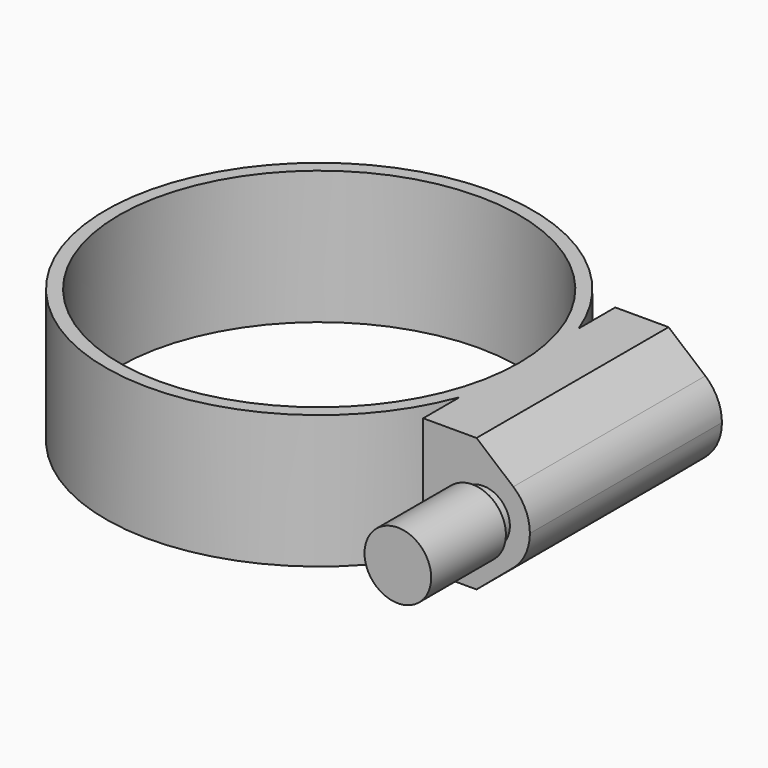
from build123d import *

# Parameters (mm, degrees)
F4_DEPTH      = 9
F4_DEPTH_BACK = 9


with BuildPart() as f3:
    # F2 (on plane+point) → F3 (revolve)
    with BuildSketch(Plane.XY.offset(5)):
        Polygon((19.5, -17), (19.5, 11), (18.5, 11), (17.5, 10), (17.5, -10), (17, -10), (17, -17), align=None)
    revolve(axis=Axis((19.5, -3, 5), (0, -1, 0)))

    # F0 (on Front) → F4 (join, two sides)
    with BuildSketch(Plane.XZ) as f4_sk:
        Polygon((15, 10), (15, 0), (16, 0), (16, 5), (16, 10), align=None)
        with BuildLine():
            Line((16, 10), (16, 5))
            ThreePointArc((16, 5), (18.024725, 8.173888), (21.756323, 7.675632))
            Line((21.756323, 7.675632), (19, 10))
            Line((19, 10), (16, 10))
        make_face()
        with BuildLine():
            Line((16, 5), (16, 0))
            Line((16, 0), (19, 0))
            Line((19, 0), (21.756323, 2.324368))
            ThreePointArc((21.756323, 2.324368), (18.024725, 1.826112), (16, 5))
        make_face()
        with BuildLine():
            ThreePointArc((21.756323, 7.675632), (18.024725, 8.173888), (16, 5))
            ThreePointArc((16, 5), (18.024725, 1.826112), (21.756323, 2.324368))
            ThreePointArc((21.756323, 2.324368), (22.673888, 3.524725), (23, 5))
            ThreePointArc((23, 5), (22.673888, 6.475275), (21.756323, 7.675632))
        make_face()
    extrude(amount=F4_DEPTH)
    extrude(f4_sk.sketch, amount=-F4_DEPTH_BACK)

    # F0 (on Front) → F5 (revolve)
    with BuildSketch(Plane.XZ):
        Polygon((15, 10), (15, 0), (16, 0), (16, 5), (16, 10), align=None)
    revolve(axis=Axis((0, 0, 5), (0, 0, 1)))


solid = f3.part
